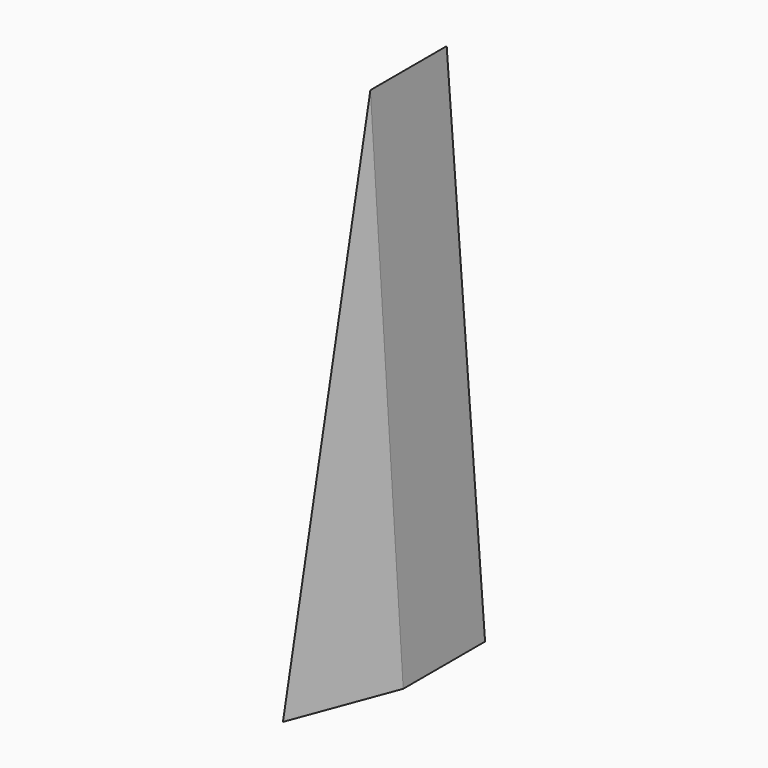
from build123d import *

# Parameters (mm, degrees)
F1_DEPTH = 100
F3_DEPTH = 35
F4_SIZE2 = 99.99999
F4_SIZE  = 7.49999


# Not quite as in the source:
# - a fillet or chamfer is up to 0.001 mm smaller than in the source, because OpenCascade refuses the exact size


with BuildPart() as f1:
    # F0 (on Top) → F1 (new body)
    with BuildSketch(Plane.XY):
        Polygon((-7.5, 20), (-7.5, 0), (0, -20), (7.5, 0), (7.5, 20), align=None)
    extrude(amount=F1_DEPTH)

    # F2 (on face) → F3 (cut)
    with BuildSketch(Plane(origin=(0, 0, 0), x_dir=(1, 0, 0), z_dir=(0, 0, -1))):
        Polygon((0, 8.6079950062), (-3.5, -0.7253383271), (-3.5, -16), (3.5, -16), (3.5, -0.7253383271), align=None)
    extrude(amount=-F3_DEPTH, mode=Mode.SUBTRACT)

    # F4 (size 7.5 and 100 in the source; OpenCascade refuses exactly that, so slightly less here)
    f4_edges = [f1.edges().sort_by_distance(p)[0] for p in [
        (3.75, -10, 100),
        (-3.75, -10, 100),
        (7.5, 10, 100),
        (-7.5, 10, 100),
    ]]
    f4_side = f1.faces().sort_by_distance((0, 4.444444, 100))[0]
    chamfer(f4_edges, length=F4_SIZE, length2=F4_SIZE2, reference=f4_side)


solid = f1.part
